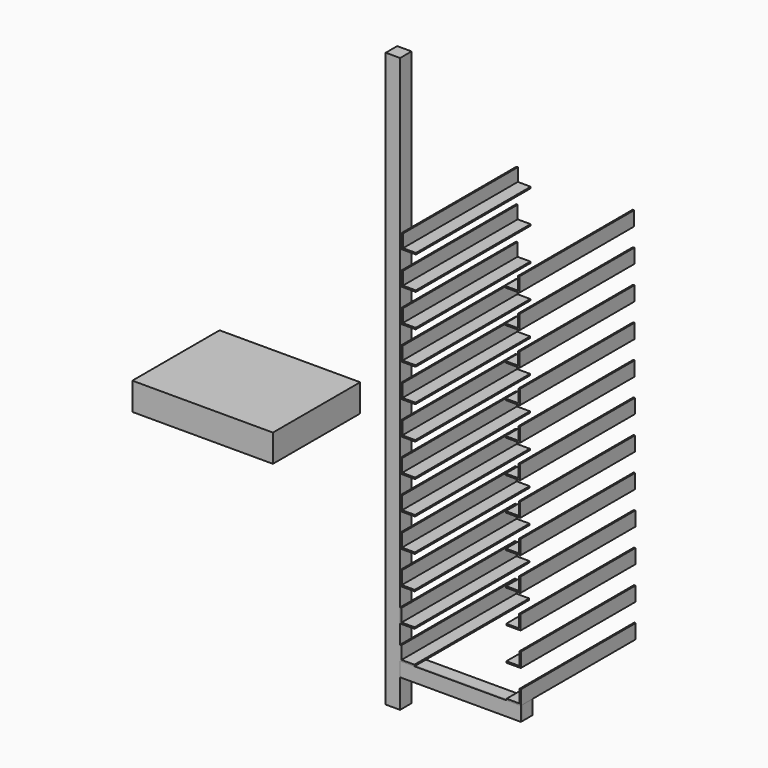
from build123d import *

# Parameters (mm, degrees)
F1_DEPTH = 500
F2_DEPTH = 50
F3_DEPTH = 5
F4_W     = 490
F4_H     = 96
F5_DEPTH = 380


with BuildPart() as f1:
    # F0 (on Front) → F1 (new body)
    with BuildSketch(Plane.XZ):
        Polygon((-618.2137493553, 1549.7096652101), (-618.2137493553, 1504.7096652101), (-663.2137493553, 1504.7096652101), (-663.2137493553, 1499.7096652101), (-613.2137493553, 1499.7096652101), (-613.2137493553, 1549.7096652101), align=None)
    extrude(amount=-F1_DEPTH)


with BuildPart() as f1b:
    # F0 (on Front) → F1, piece 2 (new body)
    with BuildSketch(Plane.XZ):
        Polygon((-611.2749996911, 1089.7137508263), (-616.2749996911, 1089.7137508263), (-616.2749996911, 1044.7137508263), (-661.2749996911, 1044.7137508263), (-661.2749996911, 1039.7137508263), (-611.2749996911, 1039.7137508263), align=None)
    extrude(amount=-F1_DEPTH)


with BuildPart() as f1c:
    # F0 (on Front) → F1, piece 3 (new body)
    with BuildSketch(Plane.XZ):
        Polygon((-662.7290619393, 1389.7106866141), (-662.7290619393, 1384.7106866142), (-612.7290619393, 1384.7106866142), (-612.7290619393, 1434.7106866142), (-617.7290619393, 1434.7106866142), (-617.7290619393, 1389.7106866142), align=None)
    extrude(amount=-F1_DEPTH)


with BuildPart() as f1d:
    # F0 (on Front) → F1, piece 4 (new body)
    with BuildSketch(Plane.XZ):
        Polygon((-612.2443745232, 1319.7117080182), (-617.2443745232, 1319.7117080182), (-617.2443745232, 1274.7117080182), (-662.2443745232, 1274.7117080182), (-662.2443745232, 1269.7117080182), (-612.2443745232, 1269.7117080182), align=None)
    extrude(amount=-F1_DEPTH)


with BuildPart() as f1e:
    # F0 (on Front) → F1, piece 5 (new body)
    with BuildSketch(Plane.XZ):
        Polygon((-611.7596871071, 1154.7127294223), (-611.7596871071, 1204.7127294223), (-616.7596871071, 1204.7127294223), (-616.7596871071, 1159.7127294223), (-661.7596871071, 1159.7127294223), (-661.7596871071, 1154.7127294223), align=None)
    extrude(amount=-F1_DEPTH)


with BuildPart() as f1f:
    # F0 (on Front) → F1, piece 6 (new body)
    with BuildSketch(Plane.XZ):
        Polygon((-659.3362500268, 584.7178364426), (-659.3362500268, 579.7178364426), (-609.3362500268, 579.7178364426), (-609.3362500268, 629.7178364426), (-614.3362500268, 629.7178364426), (-614.3362500268, 584.7178364426), align=None)
    extrude(amount=-F1_DEPTH)


with BuildPart() as f1g:
    # F0 (on Front) → F1, piece 7 (new body)
    with BuildSketch(Plane.XZ):
        Polygon((-660.305624859, 814.7157936345), (-660.305624859, 809.7157936345), (-610.305624859, 809.7157936345), (-610.305624859, 859.7157936345), (-615.305624859, 859.7157936345), (-615.305624859, 814.7157936345), align=None)
    extrude(amount=-F1_DEPTH)


with BuildPart() as f1h:
    # F0 (on Front) → F1, piece 8 (new body)
    with BuildSketch(Plane.XZ):
        Polygon((-609.8209374429, 744.7168150385), (-614.8209374429, 744.7168150385), (-614.8209374429, 699.7168150385), (-659.8209374429, 699.7168150385), (-659.8209374429, 694.7168150385), (-609.8209374429, 694.7168150385), align=None)
    extrude(amount=-F1_DEPTH)


with BuildPart() as f1i:
    # F0 (on Front) → F1, piece 9 (new body)
    with BuildSketch(Plane.XZ):
        Polygon((-658.8515626108, 469.7188578467), (-658.8515626108, 464.7188578467), (-608.8515626108, 464.7188578467), (-608.8515626108, 514.7188578467), (-613.8515626108, 514.7188578467), (-613.8515626108, 469.7188578467), align=None)
    extrude(amount=-F1_DEPTH)


with BuildPart() as f1j:
    # F0 (on Front) → F1, piece 10 (new body)
    with BuildSketch(Plane.XZ):
        Polygon((-660.790312275, 929.7147722304), (-660.790312275, 924.7147722304), (-610.790312275, 924.7147722304), (-610.790312275, 974.7147722304), (-615.790312275, 974.7147722304), (-615.790312275, 929.7147722304), align=None)
    extrude(amount=-F1_DEPTH)


with BuildPart() as f1k:
    # F0 (on Front) → F1, piece 11 (new body)
    with BuildSketch(Plane.XZ):
        Polygon((-658.3668751947, 354.7198792507), (-658.3668751947, 349.7198792507), (-608.3668751947, 349.7198792507), (-608.3668751947, 399.7198792507), (-613.3668751947, 399.7198792507), (-613.3668751947, 354.7198792507), align=None)
    extrude(amount=-F1_DEPTH)


with BuildPart() as f1l:
    # F0 (on Front) → F1, piece 12 (new body)
    with BuildSketch(Plane.XZ):
        Polygon((-1018.6178918419, 1549.7096652101), (-1023.6178918419, 1549.7096652101), (-1023.6178918419, 1499.7096652101), (-973.6178918419, 1499.7096652101), (-973.6178918419, 1504.7096652101), (-1018.6178918419, 1504.7096652101), align=None)
    extrude(amount=-F1_DEPTH)


with BuildPart() as f1m:
    # F0 (on Front) → F1, piece 13 (new body)
    with BuildSketch(Plane.XZ):
        Polygon((-1019.1025792579, 1434.7106866142), (-1024.1025792579, 1434.7106866142), (-1024.1025792579, 1384.7106866142), (-974.1025792579, 1384.7106866142), (-974.1025792579, 1389.7106866141), (-1019.1025792579, 1389.7106866142), align=None)
    extrude(amount=-F1_DEPTH)


with BuildPart() as f1n:
    # F0 (on Front) → F1, piece 14 (new body)
    with BuildSketch(Plane.XZ):
        Polygon((-1028.9494534186, 284.7209006548), (-1028.9494534186, 234.7209006548), (-978.9494534186, 234.7209006548), (-978.9494534186, 239.7209006548), (-1023.9494534186, 239.7209006548), (-1023.9494534186, 284.7209006548), align=None)
    extrude(amount=-F1_DEPTH)

    # F0 (on Front) → F2 (join)
    with BuildSketch(Plane.XZ):
        Polygon((-1078.9494534186, 2084.7209006548), (-1078.9494534186, 84.7209006548), (-1028.9494534186, 84.7209006548), (-1028.9494534186, 184.7209006548), (-1028.9494534186, 234.7209006548), (-1028.9494534186, 284.7209006548), (-1028.9494534186, 2034.7209006548), (-1028.9494534186, 2084.7209006548), align=None)
        Polygon((-1028.9494534186, 234.7209006548), (-1028.9494534186, 184.7209006548), (-607.8821877786, 184.7209006548), (-607.8821877786, 234.7209006548), (-657.8821877786, 234.7209006548), (-978.9494534186, 234.7209006548), align=None)
    extrude(amount=-F2_DEPTH)


with BuildPart() as f1o:
    # F0 (on Front) → F1, piece 15 (new body)
    with BuildSketch(Plane.XZ):
        Polygon((-1023.4647660025, 399.7198792507), (-1028.4647660025, 399.7198792507), (-1028.4647660025, 349.7198792507), (-978.4647660025, 349.7198792507), (-978.4647660025, 354.7198792507), (-1023.4647660025, 354.7198792507), align=None)
    extrude(amount=-F1_DEPTH)


with BuildPart() as f1p:
    # F0 (on Front) → F1, piece 16 (new body)
    with BuildSketch(Plane.XZ):
        Polygon((-657.8821877786, 234.7209006548), (-607.8821877786, 234.7209006548), (-607.8821877786, 284.7209006548), (-612.8821877786, 284.7209006548), (-612.8821877786, 239.7209006548), (-657.8821877786, 239.7209006548), align=None)
    extrude(amount=-F1_DEPTH)


with BuildPart() as f1q:
    # F0 (on Front) → F1, piece 17 (new body)
    with BuildSketch(Plane.XZ):
        Polygon((-1022.9800785864, 514.7188578467), (-1027.9800785864, 514.7188578467), (-1027.9800785864, 464.7188578467), (-977.9800785864, 464.7188578467), (-977.9800785864, 469.7188578467), (-1022.9800785864, 469.7188578467), align=None)
    extrude(amount=-F1_DEPTH)


with BuildPart() as f1r:
    # F0 (on Front) → F1, piece 18 (new body)
    with BuildSketch(Plane.XZ):
        Polygon((-1022.4953911704, 629.7178364426), (-1027.4953911704, 629.7178364426), (-1027.4953911704, 579.7178364426), (-977.4953911704, 579.7178364426), (-977.4953911704, 584.7178364426), (-1022.4953911704, 584.7178364426), align=None)
    extrude(amount=-F1_DEPTH)


with BuildPart() as f1s:
    # F0 (on Front) → F1, piece 19 (new body)
    with BuildSketch(Plane.XZ):
        Polygon((-1022.0107037543, 744.7168150385), (-1027.0107037543, 744.7168150385), (-1027.0107037543, 694.7168150385), (-977.0107037543, 694.7168150385), (-977.0107037543, 699.7168150385), (-1022.0107037543, 699.7168150385), align=None)
    extrude(amount=-F1_DEPTH)


with BuildPart() as f1t:
    # F0 (on Front) → F1, piece 20 (new body)
    with BuildSketch(Plane.XZ):
        Polygon((-1021.5260163382, 859.7157936345), (-1026.5260163382, 859.7157936345), (-1026.5260163382, 809.7157936345), (-976.5260163382, 809.7157936345), (-976.5260163382, 814.7157936345), (-1021.5260163382, 814.7157936345), align=None)
    extrude(amount=-F1_DEPTH)


with BuildPart() as f1u:
    # F0 (on Front) → F1, piece 21 (new body)
    with BuildSketch(Plane.XZ):
        Polygon((-1019.587266674, 1319.7117080182), (-1024.587266674, 1319.7117080182), (-1024.587266674, 1269.7117080182), (-974.587266674, 1269.7117080182), (-974.587266674, 1274.7117080182), (-1019.587266674, 1274.7117080182), align=None)
    extrude(amount=-F1_DEPTH)


with BuildPart() as f1v:
    # F0 (on Front) → F1, piece 22 (new body)
    with BuildSketch(Plane.XZ):
        Polygon((-1020.0719540901, 1204.7127294223), (-1025.0719540901, 1204.7127294223), (-1025.0719540901, 1154.7127294223), (-975.0719540901, 1154.7127294223), (-975.0719540901, 1159.7127294223), (-1020.0719540901, 1159.7127294223), align=None)
    extrude(amount=-F1_DEPTH)


with BuildPart() as f1w:
    # F0 (on Front) → F1, piece 23 (new body)
    with BuildSketch(Plane.XZ):
        Polygon((-1020.5566415061, 1089.7137508263), (-1025.5566415061, 1089.7137508263), (-1025.5566415061, 1039.7137508263), (-975.5566415061, 1039.7137508263), (-975.5566415061, 1044.7137508263), (-1020.5566415061, 1044.7137508263), align=None)
    extrude(amount=-F1_DEPTH)


with BuildPart() as f1x:
    # F0 (on Front) → F1, piece 24 (new body)
    with BuildSketch(Plane.XZ):
        Polygon((-1021.0413289222, 974.7147722304), (-1026.0413289222, 974.7147722304), (-1026.0413289222, 924.7147722304), (-976.0413289222, 924.7147722304), (-976.0413289222, 929.7147722304), (-1021.0413289222, 929.7147722304), align=None)
    extrude(amount=-F1_DEPTH)


with BuildPart() as f3:
    # F0 (on Front) → F3 (new body)
    with BuildSketch(Plane.XZ):
        Polygon((-1028.9494534186, 234.7209006548), (-1028.9494534186, 184.7209006548), (-607.8821877786, 184.7209006548), (-607.8821877786, 234.7209006548), (-657.8821877786, 234.7209006548), (-978.9494534186, 234.7209006548), align=None)
    extrude(amount=-F3_DEPTH)


with BuildPart() as f5:
    # F4 (on Front) → F5 (new body)
    with BuildSketch(Plane.XZ):
        with Locations((-1717.0861363411, 743.4093228319)):
            Rectangle(F4_W, F4_H)
    extrude(amount=-F5_DEPTH)


solid = Compound([f1.part, f1b.part, f1c.part, f1d.part, f1e.part, f1f.part, f1g.part, f1h.part, f1i.part, f1j.part, f1k.part, f1l.part, f1m.part, f1n.part, f1o.part, f1p.part, f1q.part, f1r.part, f1s.part, f1t.part, f1u.part, f1v.part, f1w.part, f1x.part, f3.part, f5.part])
